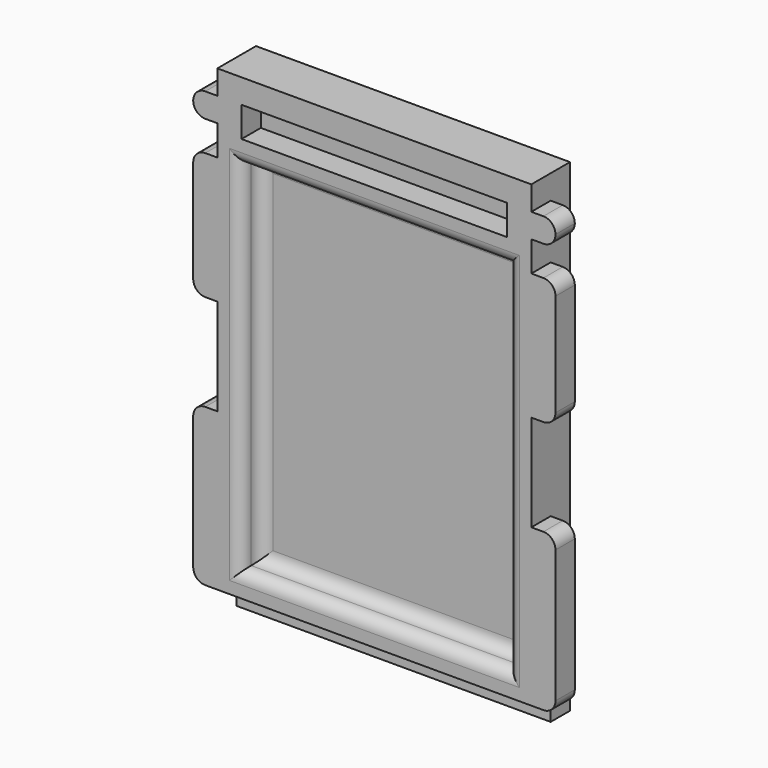
from build123d import *

# Parameters (mm, degrees)
F0_W     = 26
F0_H     = 40
F1_DEPTH = 2
F2_W     = 30
F2_H     = 40
F3_DEPTH = 2
F4_W     = 2
F4_H     = 2
F4_H_2   = 2.5
F4_W_2   = 30
F4_W_3   = 22
F4_H_3   = 8
F4_H_4   = 29.5
F5_DEPTH = 2
F6_R     = 0.99999


# Not quite as in the source:
# - a fillet or chamfer is up to 0.001 mm smaller than in the source, because OpenCascade refuses the exact size


with BuildPart() as f1:
    # F0 (on Front) → F1 (new body)
    with BuildSketch(Plane.XZ):
        with Locations((-0.059209764, 5.0314570961)):
            Rectangle(F0_W, F0_H)
    extrude(amount=F1_DEPTH)

    # F2 (on face) → F3 (join)
    with BuildSketch(Plane.XZ.offset(2)):
        with Locations((-0.059209764, 5.0314570961)):
            Rectangle(F2_W, F2_H)
    extrude(amount=F3_DEPTH)

    # F4 (on face) → F5 (cut)
    with BuildSketch(Plane.XZ.offset(4)):
        with Locations((-14.059209764, 24.0314570961)):
            Rectangle(F4_W, F4_H)
        with Locations((13.940790236, 24.0314570961)):
            Rectangle(F4_W, F4_H)
        with Locations((-14.059209764, 19.7814570961)):
            Rectangle(F4_W, F4_H_2)
        with Locations((13.940790236, 19.7814570961)):
            Rectangle(F4_W, F4_H_2)
        with Locations((-0.059209764, -13.9685429039)):
            Rectangle(F4_W_2, F4_H)
        with Locations((-0.059209764, 21.7814570961)):
            Rectangle(F4_W_3, F4_H_2)
        with Locations((-14.059209764, 4.0314570961)):
            Rectangle(F4_W, F4_H_3)
        with Locations((13.940790236, 4.0314570961)):
            Rectangle(F4_W, F4_H_3)
        with Locations((-0.059209764, 3.7814570961)):
            Rectangle(F4_W_3, F4_H_4)
    extrude(amount=-F5_DEPTH, mode=Mode.SUBTRACT)

    # F6 (radius 1 in the source; OpenCascade refuses exactly that, so slightly less here)
    f6_edges = [f1.edges().sort_by_distance(p)[0] for p in [
        (14.94079, -3, 23.031457),
        (14.94079, -3, 21.031457),
        (14.94079, -3, 18.531457),
        (14.94079, -3, -12.968543),
        (-15.05921, -3, -12.968543),
        (-15.05921, -3, 18.531457),
        (-15.05921, -3, 23.031457),
        (-15.05921, -3, 21.031457),
        (-15.05921, -3, 8.031457),
        (-15.05921, -3, 0.031457),
        (14.94079, -3, 8.031457),
        (14.94079, -3, 0.031457),
        (-0.05921, -2, -10.968543),
        (10.94079, -2, 3.781457),
        (-0.05921, -2, 18.531457),
        (-11.05921, -2, 3.781457),
        (-0.05921, -4, 18.531457),
        (-11.05921, -4, 3.781457),
        (-0.05921, -4, -10.968543),
        (10.94079, -4, 3.781457),
    ]]
    fillet(f6_edges, radius=F6_R)


solid = f1.part
